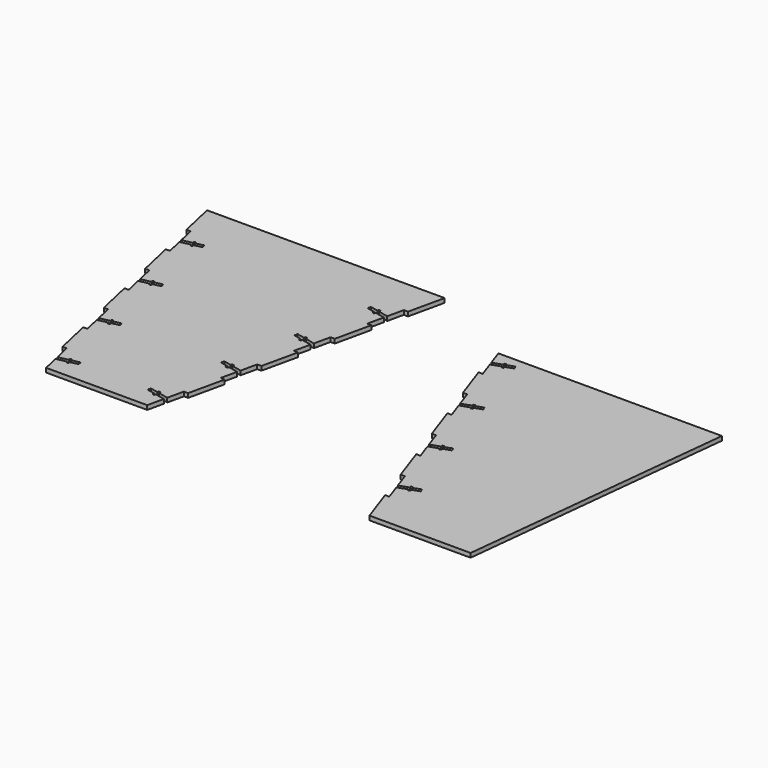
from build123d import *

# Parameters (mm, degrees)
F1_DEPTH = 3.175


# Not quite as in the source:
# - ends of sketch curves that miss each other by under 0.0002 mm in the source are joined


with BuildPart() as f1:
    # F0 (on Top) → F1 (new body)
    with BuildSketch(Plane.XY):
        Polygon((-4.6331430502, 36.5619704102), (-1.8939911218, 24.307635561), (74.3060088782, 24.307635561), (77.0451608066, 36.5619704102), (69.6086750806, 38.2242219096), (69.3290970709, 36.9853662776), (67.7185983772, 37.3488149778), (67.9974344202, 38.5843659181), (62.1721872682, 39.886462926), (62.4492291847, 41.1258772137), (62.7262711013, 42.3652915013), (68.5515182533, 41.0631944934), (68.8252918625, 42.2998770218), (70.4372635786, 41.943018245), (70.1627568273, 40.7030400019), (77.5992425538, 39.0407885023), (80.3384303136, 51.2951379635), (83.5134303136, 51.2951379635), (89.5458512708, 78.2826379635), (86.3708512708, 78.2826379635), (89.110008961, 90.5369741923), (81.673523235, 92.1992256917), (81.3939452253, 90.9603700597), (79.7834465317, 91.3238187599), (80.0622825746, 92.5593697002), (74.2370354226, 93.8614667081), (74.5140773392, 95.1008809957), (74.7911192557, 96.3402952834), (80.6163664077, 95.0381982755), (80.890140017, 96.2748808039), (82.502111733, 95.9180220271), (82.2276049817, 94.678043784), (89.6640907082, 93.0157922844), (92.4032730507, 105.270142097), (95.5782730507, 105.270142097), (101.6106940078, 132.257642097), (98.4356940078, 132.257642097), (101.1748571154, 144.5119779744), (93.7383713895, 146.1742294738), (93.4587933797, 144.9353738417), (91.8482946861, 145.2988225419), (92.127130729, 146.5343734823), (86.301883577, 147.8364704902), (86.5789254936, 149.0758847778), (86.8559674101, 150.3152990655), (92.6812145622, 149.0132020576), (92.9549881714, 150.2498845859), (94.5669598875, 149.8930258092), (94.2924531361, 148.6530475661), (101.7289388626, 146.9907960665), (104.4681157506, 159.2451460441), (107.6431157506, 159.2451460441), (113.6755367078, 186.2326460441), (110.5005367078, 186.2326460441), (113.2397052698, 198.4869817564), (105.8032195439, 200.1492332559), (105.5236415342, 198.9103776238), (103.9131428405, 199.273826324), (104.1919788834, 200.5093772644), (98.3667317314, 201.8114742722), (98.643773648, 203.0508885599), (98.9208155645, 204.2903028476), (104.7460627166, 202.9882058397), (105.0198363258, 204.224888368), (106.6318080419, 203.8680295913), (106.3573012905, 202.6280513481), (113.793787017, 200.9657998486), (116.532955579, 213.2201355609), (119.707955579, 213.2201355609), (125.7403765357, 240.207635561), (-53.3283587793, 240.207635561), (-47.2959378226, 213.2201355609), (-44.1209378226, 213.2201355609), (-41.3817692606, 200.9657998486), (-33.9452835341, 202.6280513481), (-34.2197902855, 203.8680295913), (-32.6078185694, 204.224888368), (-32.3340449601, 202.9882058397), (-26.5087978081, 204.2903028476), (-26.2317558916, 203.0508885599), (-25.954713975, 201.8114742722), (-31.779961127, 200.5093772644), (-31.5011250841, 199.273826324), (-33.1116237777, 198.9103776238), (-33.391199701, 200.1492227728), (-40.8276875134, 198.4869817564), (-38.0885189514, 186.2326460441), (-41.2635189514, 186.2326460441), (-35.2310979942, 159.2451460441), (-32.0560979942, 159.2451460441), (-29.3169211062, 146.9907960665), (-21.8804353797, 148.6530475661), (-22.154942131, 149.8930258092), (-20.542970415, 150.2498845859), (-20.2691968057, 149.0132020576), (-14.4439496537, 150.3152990655), (-14.1669077372, 149.0758847778), (-13.8898658206, 147.8364704902), (-19.7151129726, 146.5343734823), (-19.4362769297, 145.2988225419), (-21.0467756233, 144.9353738417), (-21.3263515466, 146.1742189907), (-28.762839359, 144.5119779744), (-26.0236762514, 132.257642097), (-29.1986762514, 132.257642097), (-23.1662552942, 105.270142097), (-19.9912552942, 105.270142097), (-17.2520729518, 93.0157922844), (-9.8155872253, 94.678043784), (-10.0900939766, 95.9180220271), (-8.4781222605, 96.2748808039), (-8.2043486513, 95.0381982755), (-2.3791014993, 96.3402952834), (-2.1020595827, 95.1008809957), (-1.8250176662, 93.8614667081), (-7.6502648182, 92.5593697002), (-7.3714287752, 91.3238187599), (-8.9819274689, 90.9603700597), (-9.2615033921, 92.1992152086), (-16.6979912046, 90.5369741923), (-13.9588335143, 78.2826379635), (-17.1338335143, 78.2826379635), (-11.1014125572, 51.2951379635), (-7.9264125572, 51.2951379635), (-5.1872247974, 39.0407885023), (2.2492609291, 40.7030400019), (1.9747541778, 41.943018245), (3.5867258939, 42.2998770218), (3.8604995031, 41.0631944934), (9.6857466551, 42.3652915013), (9.9627885717, 41.1258772137), (10.2398304882, 39.886462926), (4.4145833362, 38.5843659181), (4.6934193792, 37.3488149778), (3.0829206855, 36.9853662776), (2.8033447623, 38.2242114266), align=None)
    extrude(amount=F1_DEPTH)


with BuildPart() as f1b:
    # F0 (on Top) → F1, piece 2 (new body)
    with BuildSketch(Plane.XY):
        Polygon((255.1967932846, 22.2092284731), (264.336668028, -3.8901568194), (340.536668028, -3.8901568194), (362.8504252926, 204.90492552), (194.3926700813, 204.90492552), (198.5428541742, 193.0538600823), (205.7346174252, 195.5723797548), (205.3148641465, 196.7710069633), (206.8730795176, 197.3166862257), (207.2928327963, 196.1180590172), (212.9263806763, 198.0908994273), (213.346133955, 196.8922722188), (213.7658872338, 195.6936450103), (208.1323393538, 193.7208046002), (208.5520926325, 192.5221773917), (206.9938772615, 191.9764981293), (206.5741239827, 193.1751253378), (199.3823607208, 190.6566056962), (203.5325448246, 178.8055402276), (200.3575448246, 178.8055402276), (209.4974195679, 152.7061549352), (212.6724195679, 152.7061549352), (216.8226036609, 140.8550894975), (224.0143669119, 143.37360917), (223.5946136332, 144.5722363785), (225.1528290042, 145.1179156408), (225.572582283, 143.9192884323), (231.206130163, 145.8921288424), (231.6258834417, 144.6935016339), (232.0456407206, 143.4948758262), (226.4120928406, 141.5220354161), (226.8318461193, 140.3234082076), (225.2736307483, 139.7777289452), (224.8538774695, 140.9763561538), (217.6621102075, 138.4578351114), (221.8122943113, 126.6067696428), (218.6372943113, 126.6067696428), (227.7771690546, 100.5073843503), (230.9521690546, 100.5073843503), (235.1023611477, 88.6563217143), (242.2941243988, 91.1748413867), (241.87437112, 92.3734685953), (243.4325864911, 92.9191478576), (243.8523397699, 91.7205206491), (249.4858876499, 93.6933610592), (249.9056409286, 92.4947338507), (250.3253942074, 91.2961066422), (244.6918463274, 89.3232662321), (245.1115996061, 88.1246390236), (243.553384235, 87.5789597612), (243.1336309563, 88.7775869697), (235.9418676183, 86.2590673015), (240.0920437979, 74.4079990579), (236.9170437979, 74.4079990579), (246.0569185413, 48.3086137655), (249.2319185413, 48.3086137655), (253.3821146345, 36.4575525302), (260.5738778856, 38.9760722027), (260.1541246068, 40.1746994112), (261.7123399779, 40.7203786736), (262.1320932566, 39.5217514651), (267.7656411366, 41.4945918752), (268.1853944154, 40.2959646667), (268.6051476941, 39.0973374582), (262.9715998141, 37.124497048), (263.3913530929, 35.9258698395), (261.8331377218, 35.3801905772), (261.4133844431, 36.5788177857), (254.2216211051, 34.0602981175), (258.3717932846, 22.2092284731), align=None)
    extrude(amount=F1_DEPTH)


solid = Compound([f1.part, f1b.part])
